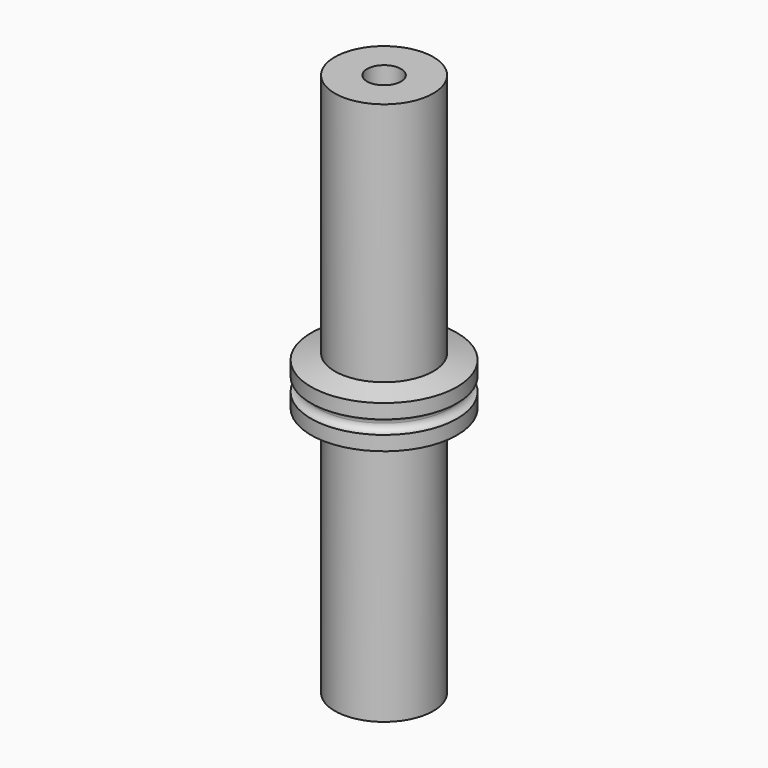
from build123d import *
from build123d import SkipClean  # not in build123d's __all__

# Parameters (mm, degrees)
F0_R        = 7.25
F0_R_2      = 2.5
F1_DEPTH    = 40
F4_S5_R     = 10.75
F4_T6_DEPTH = 17


# Not quite as in the source:
# - a fillet or chamfer that OpenCascade refuses, or shapes differently, is made with other operations: its cross-section is extruded or revolved along the edge and cut away or added


with BuildPart() as f1:
    # F0 (on Top) → F1 (new body)
    with BuildSketch(Plane.XY):
        Circle(F0_R)
        Circle(F0_R_2, mode=Mode.SUBTRACT)
    extrude(amount=F1_DEPTH)

    # F2 (on Front) → F3 (revolve)
    with BuildSketch(Plane.XZ):
        with BuildLine():
            Line((10.75, 3), (2.5, 3))
            Line((2.5, 3), (2.5, 0))
            Line((2.5, 0), (9.75, 0))
            ThreePointArc((9.75, 0), (10.0428932188, 0.7071067812), (10.75, 1))
            Line((10.75, 1), (10.75, 3))
        make_face()
    revolve(axis=Axis((0, 0, 1.5), (0, 0, 1)))

    # F4: chamfer of 4 x 1 on 1 edges, made by hand


with BuildPart() as f4_tool2:
    # F4_s3 → F4_t4 (revolve)
    with BuildSketch(Plane.XZ):
        Polygon((11.25, 3), (7.25, 4), (7.25, 3), align=None)
    revolve(axis=Axis((0, 0, 3), (0, 0, -1)))

    # F4_s5 → F4_t6 (intersect, symmetric)
    with BuildSketch(Plane.XY.offset(3.5)):
        Circle(F4_S5_R)
    extrude(amount=F4_T6_DEPTH, both=True, mode=Mode.INTERSECT)


with BuildPart() as f1_1:
    add(f1.part, clean=False)

    # F4_t1: union F4_tool2
    add(f4_tool2.part)

    # F5: F1 across face


with BuildPart() as f1_2:
    add(f1_1.part, clean=False)
    with SkipClean():  # cleaning this boolean's faces spoils the solid; the shape is the same uncleaned
        add(f1_1.part.mirror(Plane(origin=(0, 0, 0), x_dir=(1, 0, 0), z_dir=(0, 0, -1))), clean=False)


solid = f1_2.part
